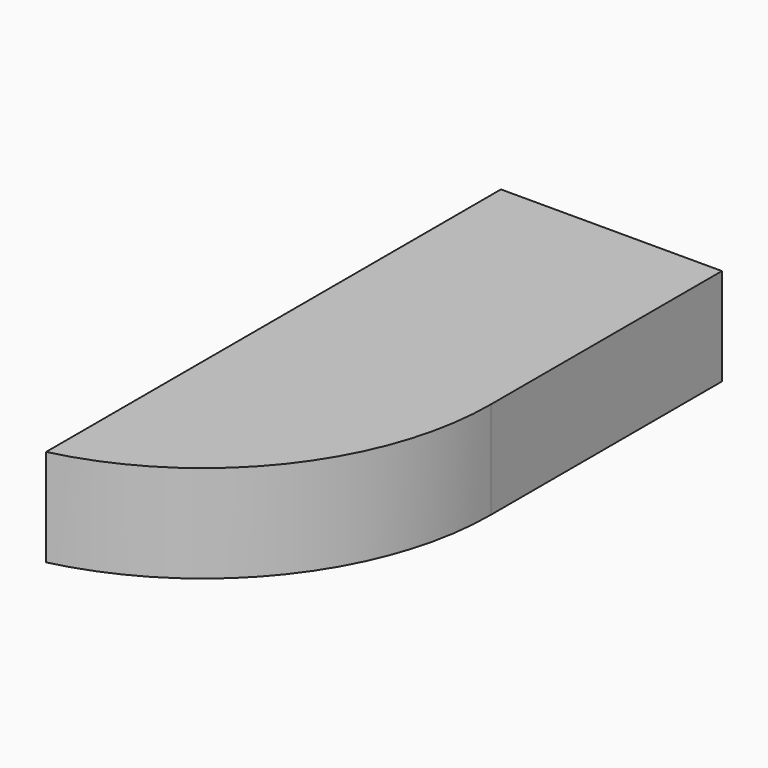
from build123d import *

# Parameters (mm, degrees)
F0_W        = 64.4432008266
F0_H        = 28.3581223339
F1_DEPTH    = 165.79635
F2_T1_DEPTH = 436.6148273869


# Not quite as in the source:
# - a fillet or chamfer that OpenCascade refuses, or shapes differently, is made with other operations: its cross-section is extruded or revolved along the edge and cut away or added


with BuildPart() as f1:
    # F0 (on Front) → F1 (new body)
    with BuildSketch(Plane.XZ):
        Rectangle(F0_W, F0_H)
    extrude(amount=F1_DEPTH)

    # F2: fillet of radius 83.9488687931 on 1 edges, made by hand

    # F2_s2 → F2_t1 (cut)
    with BuildSketch(Plane.XY.offset(-218.3074136934)):
        with BuildLine():
            ThreePointArc((32.2216004133, -84.1450089894), (14.1699672697, -136.1543053258), (-32.2216004133, -165.79635))
            Line((-32.2216004133, -165.79635), (32.2216004133, -165.79635))
            Line((32.2216004133, -165.79635), (32.2216004133, -84.1450089894))
        make_face()
    extrude(amount=F2_T1_DEPTH, mode=Mode.SUBTRACT)


solid = f1.part
